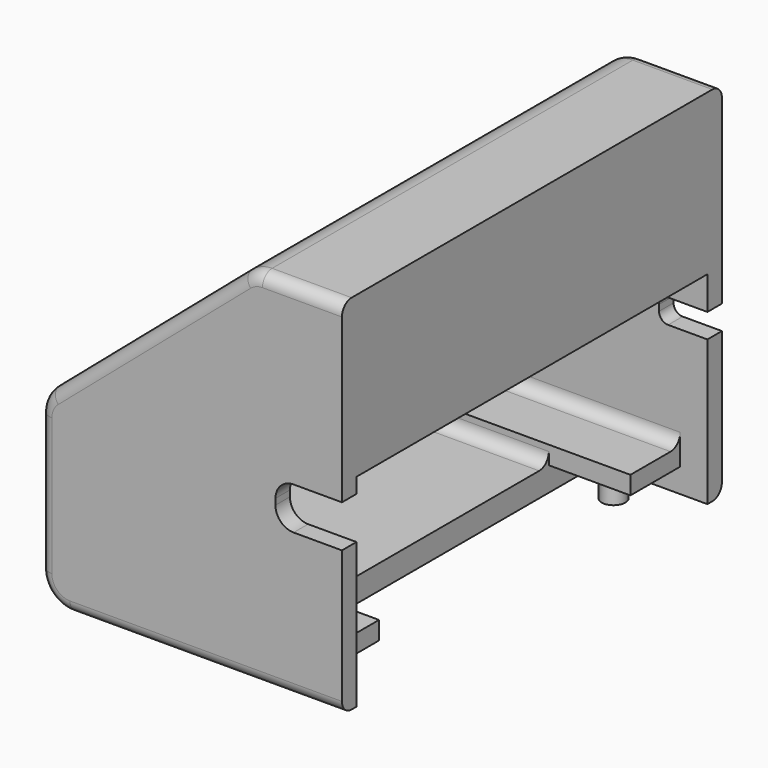
from build123d import *

# Parameters (mm, degrees)
F1_DEPTH  = 78.6
F4_DEPTH  = 72.6
F5_W      = 18
F5_H      = 72.6
F6_DEPTH  = 5
F8_DEPTH  = 5
F10_DEPTH = 5
F11_R     = 5
F12_R     = 2
F13_W     = 10.3
F13_H     = 3
F14_DEPTH = 42.5
F16_R     = 1.95
F17_DEPTH = 4
F18_SIZE  = 2
F19_R     = 2


with BuildPart() as f1:
    # F0 (on Front) → F1 (new body)
    with BuildSketch(Plane.XZ):
        Polygon((-50, 0), (0, 0), (0, 60), (-15, 60), (-50, 30), align=None)
    extrude(amount=F1_DEPTH)

    # F3 (on offset) → F4 (cut)
    with BuildSketch(Plane.XZ.offset(3)):
        Polygon((-47, 4), (0, 4), (0, 33.5), (-3, 33.5), (-3, 54), (-17.3902277714, 54), (-47, 28.6201952326), align=None)
    extrude(amount=F4_DEPTH, mode=Mode.SUBTRACT)

    # F5 (on face) → F6 (cut)
    with BuildSketch(Plane(origin=(0, 0, 0), x_dir=(1, 0, 0), z_dir=(0, 0, -1))):
        with Locations((-9, 39.3)):
            Rectangle(F5_W, F5_H)
    extrude(amount=-F6_DEPTH, mode=Mode.SUBTRACT)

    # F7 (on Front) → F8 (cut)
    with BuildSketch(Plane.XZ):
        with BuildLine():
            Line((-6.5, 24), (0, 24))
            Line((0, 24), (0, 28))
            Line((0, 28), (-6.5, 28))
            ThreePointArc((-6.5, 28), (-7.5606601718, 27.5606601718), (-8, 26.5))
            Line((-8, 26.5), (-8, 25.5))
            ThreePointArc((-8, 25.5), (-7.5606601718, 24.4393398282), (-6.5, 24))
        make_face()
    extrude(amount=F8_DEPTH, mode=Mode.SUBTRACT)

    # F9 (on face) → F10 (cut)
    with BuildSketch(Plane.XZ.offset(78.6)):
        with BuildLine():
            Line((-8, 24), (0, 24))
            Line((0, 24), (0, 31))
            Line((0, 31), (-8, 31))
            ThreePointArc((-8, 31), (-10.1213203436, 30.1213203436), (-11, 28))
            Line((-11, 28), (-11, 27))
            ThreePointArc((-11, 27), (-10.1213203436, 24.8786796564), (-8, 24))
        make_face()
    extrude(amount=-F10_DEPTH, mode=Mode.SUBTRACT)

    # F11
    f11_edges = [f1.edges().sort_by_distance(p)[0] for p in [
        (-15, -39.3, 60),
        (-50, -39.3, 30),
        (-50, -39.3, 0),
    ]]
    fillet(f11_edges, radius=F11_R)

    # F12
    f12_edges = [f1.edges().sort_by_distance(p)[0] for p in [
        (-32.329147, 0, 45.146446),
        (-32.329147, -78.6, 45.146446),
        (-22.5, 0, 0),
        (-22.5, -78.6, 0),
        (-50, 0, 16.350163),
        (-49.542564, 0, 29.789609),
        (-48.535534, 0, 1.464466),
        (-14.885111, 0, 59.689425),
        (-6.57519, 0, 60),
        (-48.535534, -78.6, 1.464466),
        (-50, -78.6, 16.350163),
        (-49.542564, -78.6, 29.789609),
        (-14.885111, -78.6, 59.689425),
        (-6.57519, -78.6, 60),
        (-10.195114, -3, 54),
        (-32.195114, -3, 41.310098),
        (-47, -3, 16.310098),
        (-47, -75.6, 16.310098),
        (-32.195114, -75.6, 41.310098),
        (-10.195114, -75.6, 54),
        (-17.390228, -39.3, 54),
        (-47, -39.3, 28.620195),
    ]]
    fillet(f12_edges, radius=F12_R)

    # F13 (on face) → F14 (join)
    with BuildSketch(Plane.YZ.offset(-47)):
        with Locations((-8.15, 5.5)):
            Rectangle(F13_W, F13_H)
        with Locations((-70.45, 5.5)):
            Rectangle(F13_W, F13_H)
    extrude(amount=F14_DEPTH)

    # F16 (on offset) → F17 (join)
    with BuildSketch(Plane.XY.offset(4)):
        with Locations((-10.5, -9.3)):
            Circle(F16_R)
        with Locations((-10.5, -69.3)):
            Circle(F16_R)
    extrude(amount=-F17_DEPTH)

    # F18
    f18_edges = [f1.edges().sort_by_distance(p)[0] for p in [
        (-3, -39.3, 33.5),
    ]]
    chamfer(f18_edges, length=F18_SIZE)

    # F19
    f19_edges = [f1.edges().sort_by_distance(p)[0] for p in [
        (-47, -9.15, 7),
        (-47, -13.3, 5.5),
        (-47, -69.45, 7),
        (-47, -65.3, 5.5),
        (-24.75, -75.6, 7),
        (-24.75, -3, 7),
        (-46.414214, -3.585786, 7),
        (-32.5, -13.3, 4),
        (-32.5, -65.3, 4),
        (-46.414214, -75.014214, 7),
    ]]
    fillet(f19_edges, radius=F19_R)


solid = f1.part
